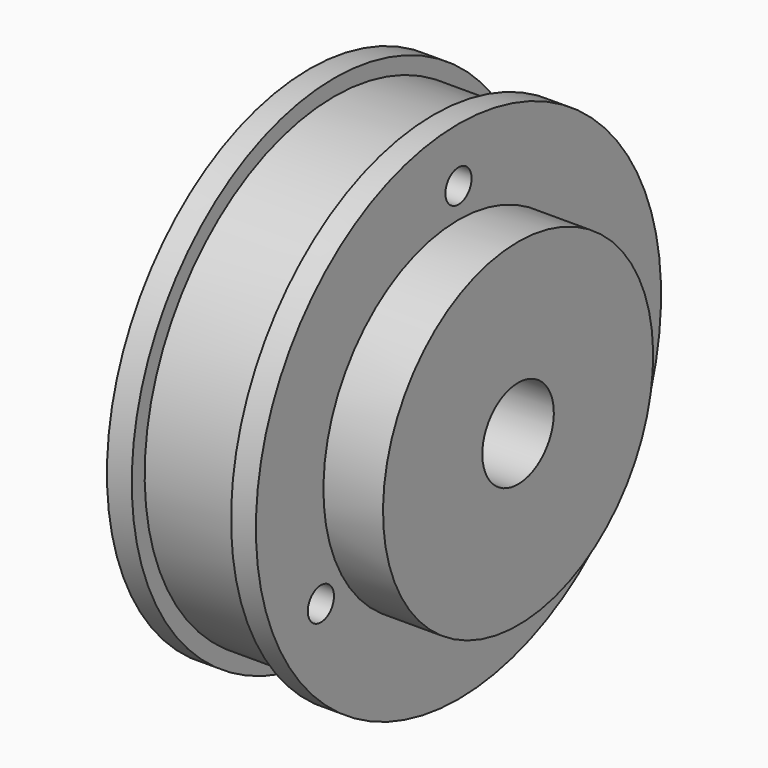
from build123d import *

# Parameters (mm, degrees)
F3_D            = 3.3
F3_CBORE_D      = 6.5
F3_CBORE_DEPTH  = 3
F3_COPIES_COUNT = 3


# Not quite as in the source:
# - a pattern or mirror of a feature is missing from the dataset's text; its kind, count and spacing are read off the source's solid


with BuildPart() as f1:
    # F0 (on Front) → F1 (revolve)
    with BuildSketch(Plane.XZ):
        Polygon((-8, 4.5), (6, 4.5), (6, 17), (0, 17), (0, 25.5), (-2.5, 25.5), (-2.5, 23.875), (-12.5, 23.875), (-12.5, 25.5), (-15, 25.5), (-15, 11), (-8, 11), align=None)
    revolve(axis=Axis((0.8759173031, 0, 0), (1, 0, 0)))

    # F3 (through all)
    with Locations(Plane(origin=(-15, 0, 0), x_dir=(0, -1, 0), z_dir=(-1, 0, 0))):
        with Locations((0, 20)):
            f3 = CounterBoreHole(F3_D / 2, F3_CBORE_D / 2, F3_CBORE_DEPTH)

    # F3_copies: F3 ×3 about axis
    f3_copies_axis = Axis((0, 0, 0), (1, 0, 0))
    for i in range(1, F3_COPIES_COUNT):
        add(f3.rotate(f3_copies_axis, i * 360 / F3_COPIES_COUNT), mode=Mode.SUBTRACT)


solid = f1.part
